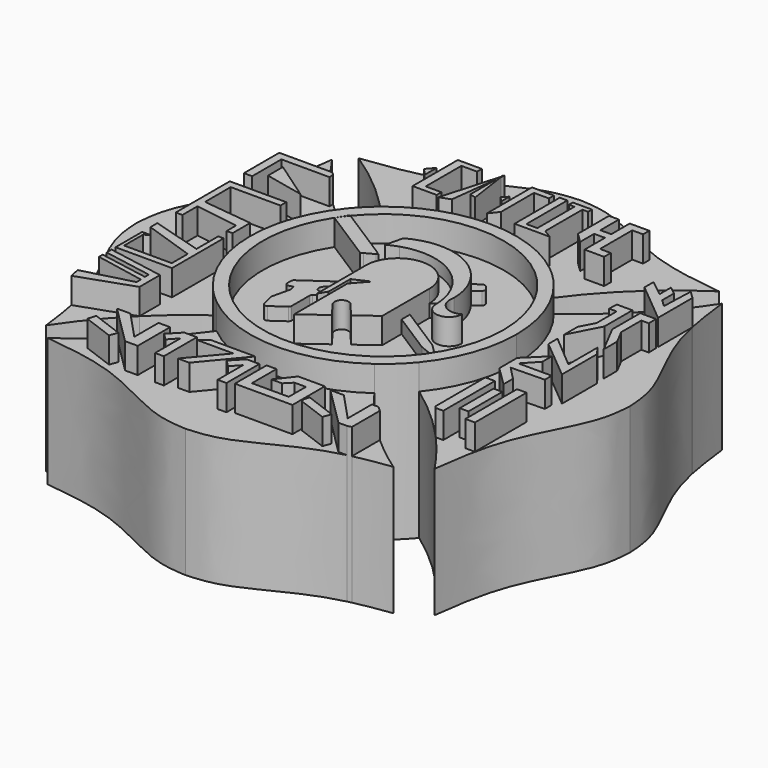
from build123d import *

# Parameters (mm, degrees)
F1_DEPTH = 25.4
F0_W     = 1.7295368016
F0_H     = 8.3469077945
F0_W_2   = 1.8799342215
F0_H_2   = 12.7083547413
F2_DEPTH = 27.94
F3_DEPTH = 30.48


with BuildPart() as f1:
    # F0 (on Top) → F1 (new body)
    with BuildSketch(Plane.XY):
        with BuildLine():
            Line((-9.5434431598, 6.2450544718), (-19.9389753342, 12.8866327357))
            ThreePointArc((-19.9389753342, 12.8866327357), (-6.7178785222, -22.7705544246), (23.7408517253, 0))
            ThreePointArc((23.7408517253, 0), (7.9342600231, 22.3757806239), (-18.437547291, 14.9560987738))
            Line((-18.437547291, 14.9560987738), (-8.1693225853, 8.3958556934))
            Line((-8.1693225853, 8.3958556934), (-7.0434035733, 7.6047051698))
            Line((-7.0434035733, 7.6047051698), (-7.338819981, 7.4440424639))
            Line((-7.338819981, 7.4440424639), (-5.8915200862, 6.5193802761))
            Line((-5.8915200862, 6.5193802761), (-5.6063739329, 6.337203889))
            ThreePointArc((-5.6063739329, 6.337203889), (-5.0978071301, 7.1900943467), (-4.4606007655, 7.951691599))
            Line((-4.4606007655, 7.951691599), (-6.14196317, 11.6369343908))
            ThreePointArc((-6.14196317, 11.6369343908), (-7.2015175666, 11.220879576), (-8.2185240178, 10.709552864))
            Line((-8.2185240178, 10.709552864), (-7.3757171631, 14.1661595553))
            ThreePointArc((-7.3757171631, 14.1661595553), (0.1389586127, 15.6738469109), (7.1075247354, 12.4828346309))
            Line((7.1075247354, 12.4828346309), (8.6497746395, 13.5536975911))
            ThreePointArc((8.6497746395, 13.5536975911), (9.0804497837, 13.6546140229), (9.4635845627, 13.4335417562))
            Line((9.4635845627, 13.4335417562), (10.0592304389, 12.6827814665))
            ThreePointArc((10.0592304389, 12.6827814665), (10.1854985957, 12.2403385238), (9.9619292605, 11.8381990487))
            Line((9.9619292605, 11.8381990487), (8.6400744323, 10.7894523474))
            ThreePointArc((8.6400744323, 10.7894523474), (10.4625836154, 7.3364011169), (11.1228358001, 3.4881327301))
            ThreePointArc((11.1228358001, 3.4881327301), (12.1514474693, 0.3059297611), (15.4842836782, 0.0290534226))
            ThreePointArc((15.4842836782, 0.0290534226), (12.8809521086, -2.5042646054), (10.2800289453, 0.0315260388))
            ThreePointArc((10.2800289453, 0.0315260388), (9.9497055154, 2.7308254028), (9.0397551795, 5.2935038865))
            Line((9.0397551795, 5.2935038865), (6.2511023134, 3.5722714383))
            Line((6.2511023134, 3.5722714383), (6.2511023134, -1.2383925481))
            Line((6.2511023134, -1.2383925481), (15.322001506, -7.0336790136))
            Line((15.322001506, -7.0336790136), (18.4107130058, -10.1001587223))
            Line((18.4107130058, -10.1001587223), (14.3876015009, -8.4962207364))
            Line((14.3876015009, -8.4962207364), (6.2511023134, -3.297910997))
            Line((6.2511023134, -3.297910997), (6.2511023134, -8.0626364797))
            Line((6.2511023134, -8.0626364797), (2.3747377821, -10.9250742877))
            Line((2.3747377821, -10.9250742877), (0, -8.0626364797))
            ThreePointArc((0, -8.0626364797), (-1.929433955, -7.8545272669), (-2.1375431679, -9.7839612218))
            Line((-2.1375431679, -9.7839612218), (0, -12.6786604524))
            Line((0, -12.6786604524), (-4.6690521418, -16.1264454246))
            Line((-4.6690521418, -16.1264454246), (-4.6690521418, -2.9718931764))
            Line((-4.6690521418, -2.9718931764), (-2.1375431679, -0.1181978878))
            Line((-2.1375431679, -0.1181978878), (-5.2554947324, -1.5450455321))
            Line((-5.2554947324, -1.5450455321), (-5.2554947324, -6.8612064933))
            Line((-5.2554947324, -6.8612064933), (-6.2511023134, -8.5651436821))
            Line((-6.2511023134, -8.5651436821), (-6.2511023134, -0.1554940756))
            Line((-6.2511023134, -0.1554940756), (-6.4565095615, -0.2993217791))
            ThreePointArc((-6.4565095615, -0.2993217791), (-6.6782063614, -0.5906114223), (-6.6898507105, -0.9564850842))
            Line((-6.6898507105, -0.9564850842), (-6.3532546104, -2.1378945595))
            ThreePointArc((-6.3532546104, -2.1378945595), (-6.3532532132, -2.467333183), (-6.5268767557, -2.7473058105))
            Line((-6.5268767557, -2.7473058105), (-9.5615380632, -5.5079116557))
            ThreePointArc((-9.5615380632, -5.5079116557), (-9.706817276, -5.7094900403), (-9.7581679001, -5.9526011428))
            Line((-9.7581679001, -5.9526011428), (-9.7581679001, -10.3816536972))
            ThreePointArc((-9.7581679001, -10.3816536972), (-9.8260924812, -10.6592385489), (-10.0145167408, -10.8740952384))
            Line((-10.0145167408, -10.8740952384), (-12.6287511028, -12.7046018453))
            ThreePointArc((-12.6287511028, -12.7046018453), (-13.1802241081, -12.7766817128), (-13.5548146017, -12.365585684))
            Line((-13.5548146017, -12.365585684), (-14.1468444432, -10.1226799809))
            ThreePointArc((-14.1468444432, -10.1226799809), (-14.1666748611, -9.9789061741), (-14.1514706229, -9.8345698165))
            Line((-14.1514706229, -9.8345698165), (-13.3251612392, -6.2401265362))
            ThreePointArc((-13.3251612392, -6.2401265362), (-13.3100853679, -6.0897110613), (-13.3330098084, -5.9402902896))
            Line((-13.3330098084, -5.9402902896), (-13.5587407276, -5.1502324641))
            Line((-13.5587407276, -5.1502324641), (-14.2865060916, -5.3581655283))
            ThreePointArc((-14.2865060916, -5.3581655283), (-14.813673449, -5.260071091), (-15.0528176735, -4.7801356982))
            Line((-15.0528176735, -4.7801356982), (-15.0528176735, -3.89823478))
            ThreePointArc((-15.0528176735, -3.89823478), (-14.9848930924, -3.6206499283), (-14.7964688328, -3.4057932388))
            Line((-14.7964688328, -3.4057932388), (-6.2511023134, 2.5777368149))
            Line((-6.2511023134, 2.5777368149), (-6.2511023134, 3.5722714383))
            ThreePointArc((-6.2511023134, 3.5722714383), (-6.228449268, 4.1039666977), (-6.1606543141, 4.6318083912))
            Line((-6.1606543141, 4.6318083912), (-7.9261528326, 5.7597637848))
            Line((-7.9261528326, 5.7597637848), (-9.0801320579, 6.4970269871))
            Line((-9.0801320579, 6.4970269871), (-9.5434431598, 6.2450544718))
        make_face()
    extrude(amount=F1_DEPTH)


with BuildPart() as f1b:
    # F0 (on Top) → F1, piece 2 (new body)
    with BuildSketch(Plane.XY):
        with BuildLine():
            ThreePointArc((-16.6267062797, 20.2924587669), (0, 26.2341617842), (16.6267062797, 20.2924587669))
            ThreePointArc((16.6267062797, 20.2924587669), (25.2329664201, 30.182800565), (35.5137959123, 38.318593055))
            add(Edge.make_bspline(
                [(35.5137959123, 38.318593055), (30.4620352986, 38.9509589957), (20.4597656889, 40.2030164693), (7.4866494732, 48.2293636919), (2.1728610161, 48.5746910392), (0, 48.7149081634)],
                knots=[0, 0, 0, 0, 0.3760666411, 0.7445958397, 0.9996624927, 0.9996624927, 0.9996624927, 0.9996624927], degree=3))
            add(Edge.make_bspline(
                [(-35.5137959123, 38.318593055), (-30.4620352986, 38.9509589957), (-20.4597656889, 40.2030164693), (-7.4866494732, 48.2293636919), (-2.1728610161, 48.5746910392), (0, 48.7149081634)],
                knots=[0, 0, 0, 0, 0.3760666411, 0.7445958397, 0.9996624927, 0.9996624927, 0.9996624927, 0.9996624927], degree=3))
            ThreePointArc((-35.5137959123, 38.318593055), (-25.2329664201, 30.182800565), (-16.6267062797, 20.2924587669))
        make_face()
        Polygon((-19.3263869733, 34.2127773911), (-18.0286001414, 35.7136428356), (-18.0286001414, 34.2127773911), (-18.0286001414, 32.7141773911), align=None, mode=Mode.SUBTRACT)
        Polygon((-15.4862534255, 39.7773832083), (-12.3972799629, 39.7773832083), (-12.3972799629, 38.6037752032), (-15.4862534255, 38.6037752032), (-15.4862534255, 34.2127773911), (-15.4862534255, 29.8217795789), (-12.3972799629, 29.8217795789), (-12.3972799629, 28.6481715739), (-17.1347092837, 28.6481715739), (-17.1347092837, 34.2127773911), (-17.1347092837, 38.6037752032), (-17.1347092837, 39.7773832083), align=None, mode=Mode.SUBTRACT)
        Polygon((-8.408809687, 39.7450013558), (-8.2768853754, 40.2063913643), (-8.3679740047, 39.4611965301), (-7.2505346718, 31.6950798014), (-8.4751974791, 32.04524516), (-8.4751974791, 38.5840027483), (-9.649637936, 28.9759213881), (-11.7087768862, 28.2037480728), (-8.4751974791, 39.5128177376), (-8.4751974791, 40.2063913643), align=None, mode=Mode.SUBTRACT)
        Polygon((-4.2724665254, 34.2127773911), (-3.2887738198, 35.2003201842), (-3.2887738198, 34.2127773911), (-3.2887738198, 33.2252345979), align=None, mode=Mode.SUBTRACT)
        Polygon((-2.5195907801, 38.5379008949), (-2.5195907801, 39.7773832083), (-1.133499667, 39.7773832083), (1.8175337464, 39.7773832083), (1.8175337464, 38.5379008949), (-1.133499667, 38.5379008949), (-1.133499667, 34.2127773911), (-1.133499667, 30.4379425943), (-2.5195907801, 28.6481715739), (-2.5195907801, 34.2127773911), align=None, mode=Mode.SUBTRACT)
        Polygon((2.9608625919, 29.696483165), (2.9608625919, 39.7773832083), (4.4449735433, 39.7773832083), (4.4449735433, 29.696483165), (6.6135358065, 29.696483165), (6.6135358065, 38.8293154538), (5.534986034, 38.8293154538), (5.534986034, 39.7773832083), (6.6135358065, 39.7773832083), (8.1796292216, 39.7773832083), (9.3080047518, 39.7773832083), (9.3080047518, 38.8293154538), (8.1796292216, 38.8293154538), (8.1796292216, 29.696483165), (9.8721999675, 28.6481715739), (8.1796292216, 28.6481715739), (6.6135358065, 28.6481715739), (4.4449735433, 28.6481715739), (2.9608625919, 28.6481715739), align=None, mode=Mode.SUBTRACT)
        Polygon((12.6640442759, 35.2156497538), (12.6640442759, 39.7773832083), (14.6210510284, 39.7773832083), (14.6210510284, 35.2156497538), (16.7559627444, 35.2156497538), (16.7559627444, 38.2401160896), (16.7559627444, 39.7773832083), (18.4757579118, 39.7773832083), (20.6106770784, 39.7773832083), (20.6106770784, 38.2401160896), (18.4757579118, 38.2401160896), (18.4757579118, 30.2934832871), (20.6106770784, 30.2934832871), (20.6106770784, 28.6481715739), (18.4757579118, 28.6481715739), (16.7559627444, 28.6481715739), (16.7559627444, 30.2934832871), (16.7559627444, 33.6737670004), (14.6210510284, 33.6737670004), (14.6210510284, 30.2341803908), (12.6640442759, 32.1318842471), (12.6640442759, 33.6737670004), align=None, mode=Mode.SUBTRACT)
    extrude(amount=F1_DEPTH)



with BuildPart() as f1c:
    # F0 (on Top) → F1, piece 3 (new body)
    with BuildSketch(Plane.XY):
        with BuildLine():
            ThreePointArc((-20.3356751091, -16.5738215983), (-26.2341617842, 0), (-20.3356751091, 16.5738215983))
            ThreePointArc((-20.3356751091, 16.5738215983), (-24.8128492339, 20.0548614406), (-28.9973442697, 23.8827496081))
            Line((-28.9973442697, 23.8827496081), (-28.9973442697, 22.9817052072))
            Line((-28.9973442697, 22.9817052072), (-38.4649895132, 22.9817052072))
            Line((-38.4649895132, 22.9817052072), (-38.4649895132, 15.7891533872))
            Line((-38.4649895132, 15.7891533872), (-40.0955304503, 15.7891533872))
            Line((-40.0955304503, 15.7891533872), (-40.0955304503, 22.9817052072))
            Line((-40.0955304503, 22.9817052072), (-40.0955304503, 24.4979433319))
            Line((-40.0955304503, 24.4979433319), (-38.4649895132, 24.4979433319))
            Line((-38.4649895132, 24.4979433319), (-29.6104829395, 24.4979433319))
            ThreePointArc((-29.6104829395, 24.4979433319), (-34.2813337884, 29.7377471459), (-38.4109179846, 35.4139189217))
            add(Edge.make_bspline(
                [(-38.4109179846, 35.4139189217), (-39.03013029, 30.3605291582), (-40.2561441291, 20.3550339017), (-48.2486906125, 7.3610662707), (-48.5801831474, 2.0463968131), (-48.7147430824, -0.1268218738)],
                knots=[0, 0, 0, 0, 0.3760666411, 0.7445958397, 0.9996624927, 0.9996624927, 0.9996624927, 0.9996624927], degree=3))
            add(Edge.make_bspline(
                [(-39.9029320846, -25.4186008721), (-40.291396554, -23.7892445191), (-42.1955076013, -17.2767114258), (-48.2097099, -7.6121819354), (-48.5688697193, -2.2993104926), (-48.7147430824, -0.1268218738)],
                knots=[0.2537440472, 0.2537440472, 0.2537440472, 0.2537440472, 0.3760666411, 0.7445958397, 0.9996624927, 0.9996624927, 0.9996624927, 0.9996624927], degree=3))
            Line((-39.9029320846, -25.4186008721), (-30.3178839386, -22.8653751711))
            Line((-30.3178839386, -22.8653751711), (-30.3178839386, -21.7938103179))
            Line((-30.3178839386, -21.7938103179), (-40.0955304503, -19.896445463))
            Line((-40.0955304503, -19.896445463), (-40.0955304503, -18.9949036293))
            Line((-40.0955304503, -18.9949036293), (-30.4072680445, -20.7157038549))
            Line((-30.4072680445, -20.7157038549), (-30.4072680445, -19.7573721554))
            Line((-30.4072680445, -19.7573721554), (-40.0955304503, -18.0365719298))
            Line((-40.0955304503, -18.0365719298), (-40.0955304503, -16.8199502901))
            Line((-40.0955304503, -16.8199502901), (-28.9663188159, -18.7966876129))
            Line((-28.9663188159, -18.7966876129), (-28.9663188159, -23.8520183066))
            ThreePointArc((-28.9663188159, -23.8520183066), (-24.7961597103, -20.0407828139), (-20.3356751091, -16.5738215983))
        make_face()
        Polygon((-39.4113734365, -15.825872908), (-40.0955304503, -15.825872908), (-40.0955304503, -14.5612113575), (-40.0955304503, -9.270174096), (-39.4113734365, -9.270174096), (-38.4338088334, -9.270174096), (-39.4113734365, -9.9116172462), (-39.4113734365, -14.5612113575), (-30.0203710794, -14.5612113575), (-30.0203710794, -10.6391225128), (-40.0955304503, -7.2353460291), (-40.0955304503, -5.5188663701), (-30.0203710794, -8.5023660779), (-30.0203710794, -3.1159945229), (-28.9663188159, -3.1159945229), (-28.9663188159, -15.825872908), (-30.0203710794, -15.825872908), align=None, mode=Mode.SUBTRACT)
        Polygon((-28.9663188159, 3.4426770708), (-28.9663188159, -0.9187736014), (-30.131842941, -0.9187736014), (-30.131842941, 1.4352052734), (-38.7795418501, 2.7206736781), (-38.7795418501, -0.9939648608), (-40.0955304503, -0.9939648608), (-40.0955304503, 2.9162935516), (-40.0955304503, 4.7210327884), (-40.0955304503, 10.8872077962), (-40.0955304503, 12.3159609338), (-38.7795418501, 12.3159609338), (-28.9663188159, 12.3159609338), (-28.9663188159, 10.8872077962), (-38.7795418501, 10.8872077962), (-38.7795418501, 4.569871897), align=None, mode=Mode.SUBTRACT)
        Polygon((-36.6944596171, 21.1480132839), (-28.9663188159, 15.7891533872), (-36.6944596171, 17.4804798862), align=None, mode=Mode.SUBTRACT)
    extrude(amount=F1_DEPTH)


with BuildPart() as f1d:
    # F0 (on Top) → F1, piece 4 (new body)
    with BuildSketch(Plane.XY):
        with BuildLine():
            ThreePointArc((-38.2774990271, -35.2107815006), (-33.9169619408, -29.2895345009), (-28.9663188159, -23.8520183066))
            Line((-28.9663188159, -23.8520183066), (-39.4506689096, -27.5013607093))
            add(Edge.make_bspline(
                [(-38.2774990271, -35.2107815006), (-38.6070013497, -32.6363948006), (-38.9448289643, -30.0626275198), (-39.4506689096, -27.5013607093)],
                knots=[0.0099947999, 0.0099947999, 0.0099947999, 0.0099947999, 0.2017045948, 0.2017045948, 0.2017045948, 0.2017045948], degree=3))
        make_face()
    extrude(amount=F1_DEPTH)


with BuildPart() as f1e:
    # F0 (on Top) → F1, piece 5 (new body)
    with BuildSketch(Plane.XY):
        with BuildLine():
            ThreePointArc((32.9154281705, -38.6499835796), (29.2232816096, -35.9310098419), (25.7146905784, -32.9789676014))
            Line((25.7146905784, -32.9789676014), (25.7146905784, -39.8764228197))
            add(Edge.make_bspline(
                [(32.9154281705, -38.6499835796), (30.5086862404, -38.968303093), (28.1053161528, -39.3335941205), (25.7146905784, -39.8764228197)],
                knots=[0.0644873221, 0.0644873221, 0.0644873221, 0.0644873221, 0.2437419627, 0.2437419627, 0.2437419627, 0.2437419627], degree=3))
        make_face()
    extrude(amount=F1_DEPTH)


with BuildPart() as f1f:
    # F0 (on Top) → F1, piece 6 (new body)
    with BuildSketch(Plane.XY):
        with BuildLine():
            ThreePointArc((20.3356751091, 16.5738215983), (24.7155885558, 8.7960745141), (26.2341617842, 0))
            ThreePointArc((26.2341617842, 0), (24.7155885558, -8.7960745141), (20.3356751091, -16.5738215983))
            ThreePointArc((20.3356751091, -16.5738215983), (26.1532390663, -21.2149239813), (31.4520317335, -26.4405031831))
            Line((31.4520317335, -26.4405031831), (31.4520317335, -14.1721851071))
            Line((31.4520317335, -14.1721851071), (33.331965955, -14.1721851071))
            Line((33.331965955, -14.1721851071), (33.331965955, -26.8805398485))
            Line((33.331965955, -26.8805398485), (31.8503183646, -26.8805398485))
            ThreePointArc((31.8503183646, -26.8805398485), (35.2187146617, -30.9262204528), (38.2774990271, -35.2107815006))
            add(Edge.make_bspline(
                [(38.2774990271, -35.2107815006), (38.9066871287, -30.2949634039), (40.2302025567, -20.4348606893), (48.2097099, -7.6121819354), (48.5688697193, -2.2993104926), (48.7147430824, -0.1268218738)],
                knots=[0.0099947999, 0.0099947999, 0.0099947999, 0.0099947999, 0.3760666411, 0.7445958397, 0.9996624927, 0.9996624927, 0.9996624927, 0.9996624927], degree=3))
            add(Edge.make_bspline(
                [(39.7814951576, 26.3571659412), (40.2034923324, 24.3406530333), (42.055934891, 17.4290048881), (48.2486906125, 7.3610662707), (48.5801831474, 2.0463968131), (48.7147430824, -0.1268218738)],
                knots=[0.2251076454, 0.2251076454, 0.2251076454, 0.2251076454, 0.3760666411, 0.7445958397, 0.9996624927, 0.9996624927, 0.9996624927, 0.9996624927], degree=3))
            Line((39.7814951576, 26.3571659412), (39.7814951576, 17.9630034724))
            Line((39.7814951576, 17.9630034724), (31.8105734624, 24.5803744653))
            Line((31.8105734624, 24.5803744653), (31.8105734624, 26.8362947861))
            ThreePointArc((31.8105734624, 26.8362947861), (26.3526094356, 21.3925542151), (20.3356751091, 16.5738215983))
        make_face()
        with Locations((35.6254874933, -20.4511656305)):
            Rectangle(F0_W, F0_H, mode=Mode.SUBTRACT)
        with Locations((38.6333837379, -20.5263624778)):
            Rectangle(F0_W_2, F0_H_2, mode=Mode.SUBTRACT)
        Polygon((35.0392975564, -14.1721851071), (31.2011621612, -10.4123166641), (31.2011621612, -6.0132703623), (35.0392975564, -2.2534056445), (35.0392975564, -4.58452095), (32.4795174132, -7.3292254349), (39.0592871885, -7.3292254349), (39.0592871885, -9.0211666068), (32.4419185239, -9.1715603014), (35.0392975564, -11.8410660764), align=None, mode=Mode.SUBTRACT)
        Polygon((32.0551983751, 0.6040969053), (32.0551983751, 2.8600209514), (38.7086647675, -2.7797854384), (38.7086647675, 4.3910338258), (40.0261200704, 2.6344248215), (40.0261200704, -6.0132703623), align=None, mode=Mode.SUBTRACT)
        Polygon((32.0020235814, 15.6471395055), (32.0551983751, 17.4550079862), (35.1392060257, 17.4550079862), (35.1392060257, 10.5691590468), (32.0020235814, 4.534069554), (32.0020235814, 7.8573563257), (33.4837888663, 10.7078714808), (33.4837888663, 15.6471395055), align=None, mode=Mode.SUBTRACT)
        Polygon((36.6812079884, 17.4550079862), (39.765215639, 17.4550079862), (39.8183904327, 15.6471395055), (38.3366251478, 15.6471395055), (38.3366251478, 10.7078714808), (39.8183904327, 7.8573563257), (39.8183904327, 4.534069554), (36.6812079884, 10.5691590468), align=None, mode=Mode.SUBTRACT)
    extrude(amount=F1_DEPTH)


with BuildPart() as f1g:
    # F0 (on Top) → F1, piece 7 (new body)
    with BuildSketch(Plane.XY):
        with BuildLine():
            ThreePointArc((38.4109179846, 35.4139189217), (35.2747322236, 30.998921866), (31.8105734624, 26.8362947861))
            Line((31.8105734624, 26.8362947861), (35.0440621115, 24.2795852134))
            Line((35.0440621115, 24.2795852134), (35.0440621115, 27.0618871907))
            Line((35.0440621115, 27.0618871907), (36.6232052185, 25.8587283203))
            Line((36.6232052185, 25.8587283203), (36.6232052185, 22.9260326484))
            Line((36.6232052185, 22.9260326484), (38.051958356, 21.5724800835))
            Line((38.051958356, 21.5724800835), (38.2775470354, 27.8890580991))
            Line((38.2775470354, 27.8890580991), (39.7547533603, 26.4857115416))
            add(Edge.make_bspline(
                [(38.4109179846, 35.4139189217), (38.7762876513, 32.4321381698), (39.141657318, 29.4503574178), (39.7547533603, 26.4857115416)],
                knots=[0, 0, 0, 0, 0.2219002144, 0.2219002144, 0.2219002144, 0.2219002144], degree=3))
        make_face()
    extrude(amount=F1_DEPTH)


with BuildPart() as f1h:
    # F0 (on Top) → F1, piece 8 (new body)
    with BuildSketch(Plane.XY):
        with BuildLine():
            Line((15.4275732894, -21.4819234181), (15.3033273432, -21.3082006924))
            ThreePointArc((15.3033273432, -21.3082006924), (-0.8341258102, -26.2208977468), (-16.6267062797, -20.2924587669))
            ThreePointArc((-16.6267062797, -20.2924587669), (-21.4138621586, -26.2442472283), (-26.8137526248, -31.6462681696))
            Line((-26.8137526248, -31.6462681696), (-24.5010119255, -31.6462681696))
            Line((-24.5010119255, -31.6462681696), (-19.1837486203, -37.3357331448))
            Line((-19.1837486203, -37.3357331448), (-19.1837486203, -31.3804053769))
            Line((-19.1837486203, -31.3804053769), (-16.8973293479, -31.3804053769))
            Line((-16.8973293479, -31.3804053769), (-16.8973293479, -39.3562905558))
            Line((-16.8973293479, -39.3562905558), (-19.3964403446, -39.3562905558))
            Line((-19.3964403446, -39.3562905558), (-26.995701496, -31.8090835655))
            ThreePointArc((-26.995701496, -31.8090835655), (-31.1314824425, -35.2251398118), (-35.5137959123, -38.318593055))
            add(Edge.make_bspline(
                [(-35.5137959123, -38.318593055), (-30.4620352986, -38.9509589957), (-20.4597656889, -40.2030164693), (-7.4866494732, -48.2293636919), (-2.1728610161, -48.5746910392), (0, -48.7149081634)],
                knots=[0, 0, 0, 0, 0.3760666411, 0.7445958397, 0.9996624927, 0.9996624927, 0.9996624927, 0.9996624927], degree=3))
            add(Edge.make_bspline(
                [(24.9123165873, -40.065583976), (23.4170540138, -40.4314467219), (17.0361868562, -42.3211530834), (7.4866494732, -48.2293636919), (2.1728610161, -48.5746910392), (0, -48.7149081634)],
                knots=[0.263808887, 0.263808887, 0.263808887, 0.263808887, 0.3760666411, 0.7445958397, 0.9996624927, 0.9996624927, 0.9996624927, 0.9996624927], degree=3))
            Line((24.9123165873, -40.065583976), (23.2155795817, -40.065583976))
            Line((23.2155795817, -40.065583976), (15.4523800735, -32.3555615898))
            Line((15.4523800735, -32.3555615898), (18.1110080008, -32.3555615898))
            Line((18.1110080008, -32.3555615898), (23.428271306, -38.045026565))
            Line((23.428271306, -38.045026565), (23.428271306, -32.0896987971))
            Line((23.428271306, -32.0896987971), (24.7429571153, -32.0896987971))
            ThreePointArc((24.7429571153, -32.0896987971), (19.8204675296, -27.0183473246), (15.4275732894, -21.4819234181))
        make_face()
        Polygon((-28.6157503724, -37.1411293745), (-28.1167414363, -35.5278660611), (-21.948726135, -37.8142862648), (-22.5347847712, -39.3952811446), align=None, mode=Mode.SUBTRACT)
        Polygon((-14.9043574929, -35.0307189029), (-16.2579119205, -33.6771644752), (-14.0771865845, -31.4212441545), (-11.5956738591, -31.4212441545), (-11.5956738591, -39.5425595444), (-13.325214386, -39.5425595444), (-13.325214386, -33.301178376), align=None, mode=Mode.SUBTRACT)
        Polygon((-7.1978791382, -38.7864187358), (-9.4538031842, -38.7864187358), (-3.8139967944, -32.1329523434), (-10.9848160587, -32.1329523434), (-9.2282070543, -30.8154970406), (-0.5805118706, -30.8154970406), align=None, mode=Mode.SUBTRACT)
        Polygon((-1.8102118192, -35.9862744808), (-3.1637662469, -34.6327200532), (-0.9830409108, -32.3767997324), (1.4984718146, -32.3767997324), (1.4984718146, -40.4981151223), (-0.2310687123, -40.4981151223), (-0.2310687123, -34.256733954), align=None, mode=Mode.SUBTRACT)
        Polygon((14.1554349825, -37.335851355), (14.49527849, -36.2371594813), (20.6632937913, -38.523579685), (20.0772351551, -40.1045745648), (14.4032866999, -38.001299889), align=None, mode=Mode.SUBTRACT)
        Polygon((2.6414692402, -39.8631114613), (2.6414692402, -32.0426062781), (4.5965984464, -32.0426062781), (4.5965984464, -38.0959943969), (11.8531472981, -38.0959943969), (11.8531472981, -33.8699700235), (9.5842894095, -33.8699700235), (8.2436725497, -35.2384937096), (6.1381459236, -35.2384937096), (8.7700523436, -31.8922107208), (13.9962695539, -31.8922107208), (13.9962695539, -39.8631114613), align=None, mode=Mode.SUBTRACT)
    extrude(amount=F1_DEPTH)


with BuildPart() as f1i:
    # F0 (on Top) → F1, piece 9 (new body)
    with BuildSketch(Plane.XY):
        with BuildLine():
            add(Edge.make_bspline(
                [(-7.2091906331, -1.5097639989), (-8.2920949454, 0.046911573), (-9.9321888534, -2.2490228676), (-11.5722827613, -4.5449573081), (-8.8492845411, -3.8056984394), (-6.1262863209, -3.0664395708), (-7.2091906331, -1.5097639989)],
                knots=[0, 0, 0, 2.0943951024, 2.0943951024, 4.1887902048, 4.1887902048, 6.2831853072, 6.2831853072, 6.2831853072], degree=2, weights=[1, 0.5, 1, 0.5, 1, 0.5, 1]))
        make_face()
    extrude(amount=F1_DEPTH)

    # F0 (on Top) → F2 (join)
    with BuildSketch(Plane.XY):
        with BuildLine():
            Line((-6.2511023134, -0.1554940756), (-6.2511023134, 2.5777368149))
            Line((-6.2511023134, 2.5777368149), (-14.7964688328, -3.4057932388))
            ThreePointArc((-14.7964688328, -3.4057932388), (-14.9848930924, -3.6206499283), (-15.0528176735, -3.89823478))
            Line((-15.0528176735, -3.89823478), (-15.0528176735, -4.7801356982))
            ThreePointArc((-15.0528176735, -4.7801356982), (-14.813673449, -5.260071091), (-14.2865060916, -5.3581655283))
            Line((-14.2865060916, -5.3581655283), (-13.5587407276, -5.1502324641))
            Line((-13.5587407276, -5.1502324641), (-13.3330098084, -5.9402902896))
            ThreePointArc((-13.3330098084, -5.9402902896), (-13.3100853679, -6.0897110613), (-13.3251612392, -6.2401265362))
            Line((-13.3251612392, -6.2401265362), (-14.1514706229, -9.8345698165))
            ThreePointArc((-14.1514706229, -9.8345698165), (-14.1666748611, -9.9789061741), (-14.1468444432, -10.1226799809))
            Line((-14.1468444432, -10.1226799809), (-13.5548146017, -12.365585684))
            ThreePointArc((-13.5548146017, -12.365585684), (-13.1802241081, -12.7766817128), (-12.6287511028, -12.7046018453))
            Line((-12.6287511028, -12.7046018453), (-10.0145167408, -10.8740952384))
            ThreePointArc((-10.0145167408, -10.8740952384), (-9.8260924812, -10.6592385489), (-9.7581679001, -10.3816536972))
            Line((-9.7581679001, -10.3816536972), (-9.7581679001, -5.9526011428))
            ThreePointArc((-9.7581679001, -5.9526011428), (-9.706817276, -5.7094900403), (-9.5615380632, -5.5079116557))
            Line((-9.5615380632, -5.5079116557), (-6.5268767557, -2.7473058105))
            ThreePointArc((-6.5268767557, -2.7473058105), (-6.3532532132, -2.467333183), (-6.3532546104, -2.1378945595))
            Line((-6.3532546104, -2.1378945595), (-6.6898507105, -0.9564850842))
            ThreePointArc((-6.6898507105, -0.9564850842), (-6.6782063614, -0.5906114223), (-6.4565095615, -0.2993217791))
            Line((-6.4565095615, -0.2993217791), (-6.2511023134, -0.1554940756))
        make_face()
        with BuildLine():
            add(Edge.make_bspline(
                [(-7.2091906331, -1.5097639989), (-8.2920949454, 0.046911573), (-9.9321888534, -2.2490228676), (-11.5722827613, -4.5449573081), (-8.8492845411, -3.8056984394), (-6.1262863209, -3.0664395708), (-7.2091906331, -1.5097639989)],
                knots=[0, 0, 0, 2.0943951024, 2.0943951024, 4.1887902048, 4.1887902048, 6.2831853072, 6.2831853072, 6.2831853072], degree=2, weights=[1, 0.5, 1, 0.5, 1, 0.5, 1]))
        make_face(mode=Mode.SUBTRACT)
    extrude(amount=F2_DEPTH)



with BuildPart() as f2:
    # F0 (on Top) → F2, piece 2 (new body)
    with BuildSketch(Plane.XY):
        with BuildLine():
            Line((-7.338819981, 7.4440424639), (-9.0801320579, 6.4970269871))
            Line((-9.0801320579, 6.4970269871), (-7.9261528326, 5.7597637848))
            Line((-7.9261528326, 5.7597637848), (-6.1606543141, 4.6318083912))
            ThreePointArc((-6.1606543141, 4.6318083912), (-5.9449837588, 5.5044847392), (-5.6063739329, 6.337203889))
            Line((-5.6063739329, 6.337203889), (-5.8915200862, 6.5193802761))
            Line((-5.8915200862, 6.5193802761), (-7.338819981, 7.4440424639))
        make_face()
    extrude(amount=F2_DEPTH)


with BuildPart() as f2b:
    # F0 (on Top) → F2, piece 3 (new body)
    with BuildSketch(Plane.XY):
        Polygon((15.322001506, -7.0336790136), (6.2511023134, -1.2383925481), (6.2511023134, -3.297910997), (14.3876015009, -8.4962207364), (18.4107130058, -10.1001587223), align=None)
    extrude(amount=F2_DEPTH)


with BuildPart() as f2c:
    # F0 (on Top) → F2, piece 4 (new body)
    with BuildSketch(Plane.XY):
        with BuildLine():
            Line((-6.14196317, 11.6369343908), (-4.4606007655, 7.951691599))
            ThreePointArc((-4.4606007655, 7.951691599), (2.3656509007, 9.3584598165), (6.2511023134, 3.5722714383))
            Line((6.2511023134, 3.5722714383), (9.0397551795, 5.2935038865))
            ThreePointArc((9.0397551795, 5.2935038865), (2.6501831797, 11.3402571067), (-6.14196317, 11.6369343908))
        make_face()
    extrude(amount=F2_DEPTH)


with BuildPart() as f2d:
    # F0 (on Top) → F2, piece 5 (new body)
    with BuildSketch(Plane.XY):
        with BuildLine():
            Line((8.6497746395, 13.5536975911), (7.1075247354, 12.4828346309))
            ThreePointArc((7.1075247354, 12.4828346309), (7.9128114811, 11.6714501485), (8.6400744323, 10.7894523474))
            Line((8.6400744323, 10.7894523474), (9.9619292605, 11.8381990487))
            ThreePointArc((9.9619292605, 11.8381990487), (10.1854985957, 12.2403385238), (10.0592304389, 12.6827814665))
            Line((10.0592304389, 12.6827814665), (9.4635845627, 13.4335417562))
            ThreePointArc((9.4635845627, 13.4335417562), (9.0804497837, 13.6546140229), (8.6497746395, 13.5536975911))
        make_face()
    extrude(amount=F2_DEPTH)


with BuildPart() as f1i_1:
    add(f1i.part)

    add(f2.part)  # F3 merges F2

    add(f2b.part)  # F3 merges F2b

    add(f2c.part)  # F3 merges F2c
    # F0 (on Top) → F3 (join)
    with BuildSketch(Plane.XY):
        with BuildLine():
            ThreePointArc((-18.437547291, 14.9560987738), (-19.2161402113, 13.9415923057), (-19.9389753342, 12.8866327357))
            Line((-19.9389753342, 12.8866327357), (-9.5434431598, 6.2450544718))
            Line((-9.5434431598, 6.2450544718), (-8.1693225853, 8.3958556934))
            Line((-8.1693225853, 8.3958556934), (-18.437547291, 14.9560987738))
        make_face()
        Polygon((-8.1693225853, 8.3958556934), (-9.5434431598, 6.2450544718), (-9.0801320579, 6.4970269871), (-7.338819981, 7.4440424639), (-7.0434035733, 7.6047051698), align=None)
        with BuildLine():
            ThreePointArc((-5.6063739329, 6.337203889), (-5.9449837588, 5.5044847392), (-6.1606543141, 4.6318083912))
            ThreePointArc((-6.1606543141, 4.6318083912), (-6.228449268, 4.1039666977), (-6.2511023134, 3.5722714383))
            Line((-6.2511023134, 3.5722714383), (-6.2511023134, 2.5777368149))
            Line((-6.2511023134, 2.5777368149), (-6.2511023134, -0.1554940756))
            Line((-6.2511023134, -0.1554940756), (-6.2511023134, -8.5651436821))
            Line((-6.2511023134, -8.5651436821), (-5.2554947324, -6.8612064933))
            Line((-5.2554947324, -6.8612064933), (-5.2554947324, -1.5450455321))
            Line((-5.2554947324, -1.5450455321), (-2.1375431679, -0.1181978878))
            Line((-2.1375431679, -0.1181978878), (-4.6690521418, -2.9718931764))
            Line((-4.6690521418, -2.9718931764), (-4.6690521418, -16.1264454246))
            Line((-4.6690521418, -16.1264454246), (0, -12.6786604524))
            Line((0, -12.6786604524), (-2.1375431679, -9.7839612218))
            ThreePointArc((-2.1375431679, -9.7839612218), (-1.929433955, -7.8545272669), (0, -8.0626364797))
            Line((0, -8.0626364797), (2.3747377821, -10.9250742877))
            Line((2.3747377821, -10.9250742877), (6.2511023134, -8.0626364797))
            Line((6.2511023134, -8.0626364797), (6.2511023134, -3.297910997))
            Line((6.2511023134, -3.297910997), (6.2511023134, -1.2383925481))
            Line((6.2511023134, -1.2383925481), (6.2511023134, 3.5722714383))
            ThreePointArc((6.2511023134, 3.5722714383), (2.3656509007, 9.3584598165), (-4.4606007655, 7.951691599))
            ThreePointArc((-4.4606007655, 7.951691599), (-5.0978071301, 7.1900943467), (-5.6063739329, 6.337203889))
        make_face()
        with BuildLine():
            ThreePointArc((-8.2185240178, 10.709552864), (-7.2015175666, 11.220879576), (-6.14196317, 11.6369343908))
            ThreePointArc((-6.14196317, 11.6369343908), (2.6501831797, 11.3402571067), (9.0397551795, 5.2935038865))
            ThreePointArc((9.0397551795, 5.2935038865), (9.9497055154, 2.7308254028), (10.2800289453, 0.0315260388))
            ThreePointArc((10.2800289453, 0.0315260388), (12.8809521086, -2.5042646054), (15.4842836782, 0.0290534226))
            ThreePointArc((15.4842836782, 0.0290534226), (12.1514474693, 0.3059297611), (11.1228358001, 3.4881327301))
            ThreePointArc((11.1228358001, 3.4881327301), (10.4625836154, 7.3364011169), (8.6400744323, 10.7894523474))
            ThreePointArc((8.6400744323, 10.7894523474), (7.9128114811, 11.6714501485), (7.1075247354, 12.4828346309))
            ThreePointArc((7.1075247354, 12.4828346309), (0.1389586127, 15.6738469109), (-7.3757171631, 14.1661595553))
            Line((-7.3757171631, 14.1661595553), (-8.2185240178, 10.709552864))
        make_face()
    extrude(amount=F3_DEPTH)


with BuildPart() as f1b_1:
    add(f1b.part)

    add(f1c.part)  # F3#2 merges F1c

    add(f1d.part)  # F3#2 merges F1d

    add(f1e.part)  # F3#2 merges F1e

    add(f1f.part)  # F3#2 merges F1f

    add(f1g.part)  # F3#2 merges F1g

    add(f1h.part)  # F3#2 merges F1h
    # F0 (on Top) → F3, piece 2 (join)
    with BuildSketch(Plane.XY):
        with BuildLine():
            Line((-28.9973442697, 22.9817052072), (-28.9973442697, 23.8827496081))
            ThreePointArc((-28.9973442697, 23.8827496081), (-29.3048560825, 24.1894071405), (-29.6104829395, 24.4979433319))
            Line((-29.6104829395, 24.4979433319), (-38.4649895132, 24.4979433319))
            Line((-38.4649895132, 24.4979433319), (-40.0955304503, 24.4979433319))
            Line((-40.0955304503, 24.4979433319), (-40.0955304503, 22.9817052072))
            Line((-40.0955304503, 22.9817052072), (-40.0955304503, 15.7891533872))
            Line((-40.0955304503, 15.7891533872), (-38.4649895132, 15.7891533872))
            Line((-38.4649895132, 15.7891533872), (-38.4649895132, 22.9817052072))
            Line((-38.4649895132, 22.9817052072), (-28.9973442697, 22.9817052072))
        make_face()
        Polygon((-36.6944596171, 17.4804798862), (-28.9663188159, 15.7891533872), (-36.6944596171, 21.1480132839), align=None)
        Polygon((-40.0955304503, -14.5612113575), (-40.0955304503, -15.825872908), (-39.4113734365, -15.825872908), (-30.0203710794, -15.825872908), (-28.9663188159, -15.825872908), (-28.9663188159, -3.1159945229), (-30.0203710794, -3.1159945229), (-30.0203710794, -8.5023660779), (-40.0955304503, -5.5188663701), (-40.0955304503, -7.2353460291), (-30.0203710794, -10.6391225128), (-30.0203710794, -14.5612113575), (-39.4113734365, -14.5612113575), (-39.4113734365, -9.9116172462), (-38.4338088334, -9.270174096), (-39.4113734365, -9.270174096), (-40.0955304503, -9.270174096), align=None)
        with BuildLine():
            Line((-39.4506689096, -27.5013607093), (-28.9663188159, -23.8520183066))
            Line((-28.9663188159, -23.8520183066), (-28.9663188159, -18.7966876129))
            Line((-28.9663188159, -18.7966876129), (-40.0955304503, -16.8199502901))
            Line((-40.0955304503, -16.8199502901), (-40.0955304503, -18.0365719298))
            Line((-40.0955304503, -18.0365719298), (-30.4072680445, -19.7573721554))
            Line((-30.4072680445, -19.7573721554), (-30.4072680445, -20.7157038549))
            Line((-30.4072680445, -20.7157038549), (-40.0955304503, -18.9949036293))
            Line((-40.0955304503, -18.9949036293), (-40.0955304503, -19.896445463))
            Line((-40.0955304503, -19.896445463), (-30.3178839386, -21.7938103179))
            Line((-30.3178839386, -21.7938103179), (-30.3178839386, -22.8653751711))
            Line((-30.3178839386, -22.8653751711), (-39.9029320846, -25.4186008721))
            add(Edge.make_bspline(
                [(-39.4506689096, -27.5013607093), (-39.5879787104, -26.8061071244), (-39.7376684354, -26.1117746319), (-39.9029320846, -25.4186008721)],
                knots=[0.2017045948, 0.2017045948, 0.2017045948, 0.2017045948, 0.2537440472, 0.2537440472, 0.2537440472, 0.2537440472], degree=3))
        make_face()
        Polygon((-30.131842941, -0.9187736014), (-28.9663188159, -0.9187736014), (-28.9663188159, 3.4426770708), (-38.7795418501, 4.569871897), (-38.7795418501, 10.8872077962), (-28.9663188159, 10.8872077962), (-28.9663188159, 12.3159609338), (-38.7795418501, 12.3159609338), (-40.0955304503, 12.3159609338), (-40.0955304503, 10.8872077962), (-40.0955304503, 4.7210327884), (-40.0955304503, 2.9162935516), (-40.0955304503, -0.9939648608), (-38.7795418501, -0.9939648608), (-38.7795418501, 2.7206736781), (-30.131842941, 1.4352052734), align=None)
        Polygon((-12.3972799629, 38.6037752032), (-12.3972799629, 39.7773832083), (-15.4862534255, 39.7773832083), (-17.1347092837, 39.7773832083), (-17.1347092837, 38.6037752032), (-17.1347092837, 34.2127773911), (-17.1347092837, 28.6481715739), (-12.3972799629, 28.6481715739), (-12.3972799629, 29.8217795789), (-15.4862534255, 29.8217795789), (-15.4862534255, 34.2127773911), (-15.4862534255, 38.6037752032), align=None)
        Polygon((-18.0286001414, 34.2127773911), (-18.0286001414, 35.7136428356), (-19.3263869733, 34.2127773911), (-18.0286001414, 32.7141773911), align=None)
        Polygon((-8.3679740047, 39.4611965301), (-8.2768853754, 40.2063913643), (-8.408809687, 39.7450013558), (-8.4751974791, 40.2063913643), (-8.4751974791, 39.5128177376), (-11.7087768862, 28.2037480728), (-9.649637936, 28.9759213881), (-8.4751974791, 38.5840027483), (-8.4751974791, 32.04524516), (-7.2505346718, 31.6950798014), align=None)
        Polygon((-1.133499667, 39.7773832083), (-2.5195907801, 39.7773832083), (-2.5195907801, 38.5379008949), (-2.5195907801, 34.2127773911), (-2.5195907801, 28.6481715739), (-1.133499667, 30.4379425943), (-1.133499667, 34.2127773911), (-1.133499667, 38.5379008949), (1.8175337464, 38.5379008949), (1.8175337464, 39.7773832083), align=None)
        Polygon((-3.2887738198, 34.2127773911), (-3.2887738198, 35.2003201842), (-4.2724665254, 34.2127773911), (-3.2887738198, 33.2252345979), align=None)
        Polygon((4.4449735433, 39.7773832083), (2.9608625919, 39.7773832083), (2.9608625919, 29.696483165), (2.9608625919, 28.6481715739), (4.4449735433, 28.6481715739), (6.6135358065, 28.6481715739), (8.1796292216, 28.6481715739), (9.8721999675, 28.6481715739), (8.1796292216, 29.696483165), (8.1796292216, 38.8293154538), (9.3080047518, 38.8293154538), (9.3080047518, 39.7773832083), (8.1796292216, 39.7773832083), (6.6135358065, 39.7773832083), (5.534986034, 39.7773832083), (5.534986034, 38.8293154538), (6.6135358065, 38.8293154538), (6.6135358065, 29.696483165), (4.4449735433, 29.696483165), align=None)
        Polygon((14.6210510284, 39.7773832083), (12.6640442759, 39.7773832083), (12.6640442759, 35.2156497538), (12.6640442759, 33.6737670004), (12.6640442759, 32.1318842471), (14.6210510284, 30.2341803908), (14.6210510284, 33.6737670004), (16.7559627444, 33.6737670004), (16.7559627444, 30.2934832871), (16.7559627444, 28.6481715739), (18.4757579118, 28.6481715739), (20.6106770784, 28.6481715739), (20.6106770784, 30.2934832871), (18.4757579118, 30.2934832871), (18.4757579118, 38.2401160896), (20.6106770784, 38.2401160896), (20.6106770784, 39.7773832083), (18.4757579118, 39.7773832083), (16.7559627444, 39.7773832083), (16.7559627444, 38.2401160896), (16.7559627444, 35.2156497538), (14.6210510284, 35.2156497538), align=None)
        with Locations((38.6333837379, -20.5263624778)):
            Rectangle(F0_W_2, F0_H_2)
        with Locations((35.6254874933, -20.4511656305)):
            Rectangle(F0_W, F0_H)
        with BuildLine():
            Line((31.4520317335, -14.1721851071), (31.4520317335, -26.4405031831))
            ThreePointArc((31.4520317335, -26.4405031831), (31.6516357073, -26.6601045641), (31.8503183646, -26.8805398485))
            Line((31.8503183646, -26.8805398485), (33.331965955, -26.8805398485))
            Line((33.331965955, -26.8805398485), (33.331965955, -14.1721851071))
            Line((33.331965955, -14.1721851071), (31.4520317335, -14.1721851071))
        make_face()
        Polygon((31.2011621612, -6.0132703623), (31.2011621612, -10.4123166641), (35.0392975564, -14.1721851071), (35.0392975564, -11.8410660764), (32.4419185239, -9.1715603014), (39.0592871885, -9.0211666068), (39.0592871885, -7.3292254349), (32.4795174132, -7.3292254349), (35.0392975564, -4.58452095), (35.0392975564, -2.2534056445), align=None)
        Polygon((38.7086647675, -2.7797854384), (32.0551983751, 2.8600209514), (32.0551983751, 0.6040969053), (40.0261200704, -6.0132703623), (40.0261200704, 2.6344248215), (38.7086647675, 4.3910338258), align=None)
        Polygon((35.1392060257, 17.4550079862), (32.0551983751, 17.4550079862), (32.0020235814, 15.6471395055), (33.4837888663, 15.6471395055), (33.4837888663, 10.7078714808), (32.0020235814, 7.8573563257), (32.0020235814, 4.534069554), (35.1392060257, 10.5691590468), align=None)
        with BuildLine():
            Line((35.0440621115, 24.2795852134), (31.8105734624, 26.8362947861))
            Line((31.8105734624, 26.8362947861), (31.8105734624, 24.5803744653))
            Line((31.8105734624, 24.5803744653), (39.7814951576, 17.9630034724))
            Line((39.7814951576, 17.9630034724), (39.7814951576, 26.3571659412))
            add(Edge.make_bspline(
                [(39.7547533603, 26.4857115416), (39.7636152861, 26.4428594109), (39.7725289692, 26.4000108602), (39.7814951576, 26.3571659412)],
                knots=[0.2219002144, 0.2219002144, 0.2219002144, 0.2219002144, 0.2251076454, 0.2251076454, 0.2251076454, 0.2251076454], degree=3))
            Line((39.7547533603, 26.4857115416), (38.2775470354, 27.8890580991))
            Line((38.2775470354, 27.8890580991), (38.051958356, 21.5724800835))
            Line((38.051958356, 21.5724800835), (36.6232052185, 22.9260326484))
            Line((36.6232052185, 22.9260326484), (36.6232052185, 25.8587283203))
            Line((36.6232052185, 25.8587283203), (35.0440621115, 27.0618871907))
            Line((35.0440621115, 27.0618871907), (35.0440621115, 24.2795852134))
        make_face()
        Polygon((39.8183904327, 15.6471395055), (39.765215639, 17.4550079862), (36.6812079884, 17.4550079862), (36.6812079884, 10.5691590468), (39.8183904327, 4.534069554), (39.8183904327, 7.8573563257), (38.3366251478, 10.7078714808), (38.3366251478, 15.6471395055), align=None)
        Polygon((-3.8139967944, -32.1329523434), (-9.4538031842, -38.7864187358), (-7.1978791382, -38.7864187358), (-0.5805118706, -30.8154970406), (-9.2282070543, -30.8154970406), (-10.9848160587, -32.1329523434), align=None)
        Polygon((-14.0771865845, -31.4212441545), (-16.2579119205, -33.6771644752), (-14.9043574929, -35.0307189029), (-13.325214386, -33.301178376), (-13.325214386, -39.5425595444), (-11.5956738591, -39.5425595444), (-11.5956738591, -31.4212441545), align=None)
        with BuildLine():
            Line((-24.5010119255, -31.6462681696), (-26.8137526248, -31.6462681696))
            ThreePointArc((-26.8137526248, -31.6462681696), (-26.9046569432, -31.7277542246), (-26.995701496, -31.8090835655))
            Line((-26.995701496, -31.8090835655), (-19.3964403446, -39.3562905558))
            Line((-19.3964403446, -39.3562905558), (-16.8973293479, -39.3562905558))
            Line((-16.8973293479, -39.3562905558), (-16.8973293479, -31.3804053769))
            Line((-16.8973293479, -31.3804053769), (-19.1837486203, -31.3804053769))
            Line((-19.1837486203, -31.3804053769), (-19.1837486203, -37.3357331448))
            Line((-19.1837486203, -37.3357331448), (-24.5010119255, -31.6462681696))
        make_face()
        Polygon((-21.948726135, -37.8142862648), (-28.1167414363, -35.5278660611), (-28.6157503724, -37.1411293745), (-22.5347847712, -39.3952811446), align=None)
        Polygon((-0.9830409108, -32.3767997324), (-3.1637662469, -34.6327200532), (-1.8102118192, -35.9862744808), (-0.2310687123, -34.256733954), (-0.2310687123, -40.4981151223), (1.4984718146, -40.4981151223), (1.4984718146, -32.3767997324), align=None)
        Polygon((4.5965984464, -32.0426062781), (2.6414692402, -32.0426062781), (2.6414692402, -39.8631114613), (13.9962695539, -39.8631114613), (13.9962695539, -31.8922107208), (8.7700523436, -31.8922107208), (6.1381459236, -35.2384937096), (8.2436725497, -35.2384937096), (9.5842894095, -33.8699700235), (11.8531472981, -33.8699700235), (11.8531472981, -38.0959943969), (4.5965984464, -38.0959943969), align=None)
        Polygon((20.6632937913, -38.523579685), (14.49527849, -36.2371594813), (14.1554349825, -37.335851355), (14.4032866999, -38.001299889), (20.0772351551, -40.1045745648), align=None)
        with BuildLine():
            ThreePointArc((25.7146905784, -32.9789676014), (25.2267577343, -32.5365909088), (24.7429571153, -32.0896987971))
            Line((24.7429571153, -32.0896987971), (23.428271306, -32.0896987971))
            Line((23.428271306, -32.0896987971), (23.428271306, -38.045026565))
            Line((23.428271306, -38.045026565), (18.1110080008, -32.3555615898))
            Line((18.1110080008, -32.3555615898), (15.4523800735, -32.3555615898))
            Line((15.4523800735, -32.3555615898), (23.2155795817, -40.065583976))
            Line((23.2155795817, -40.065583976), (24.9123165873, -40.065583976))
            add(Edge.make_bspline(
                [(25.7146905784, -39.8764228197), (25.447068484, -39.9371905765), (25.1796061039, -40.0001832375), (24.9123165873, -40.065583976)],
                knots=[0.2437419627, 0.2437419627, 0.2437419627, 0.2437419627, 0.263808887, 0.263808887, 0.263808887, 0.263808887], degree=3))
            Line((25.7146905784, -39.8764228197), (25.7146905784, -32.9789676014))
        make_face()
        with BuildLine():
            ThreePointArc((20.3356751091, -16.5738215983), (24.7155885558, -8.7960745141), (26.2341617842, 0))
            ThreePointArc((26.2341617842, 0), (24.7155885558, 8.7960745141), (20.3356751091, 16.5738215983))
            ThreePointArc((20.3356751091, 16.5738215983), (18.5744845173, 18.5261914444), (16.6267062797, 20.2924587669))
            ThreePointArc((16.6267062797, 20.2924587669), (0, 26.2341617842), (-16.6267062797, 20.2924587669))
            ThreePointArc((-16.6267062797, 20.2924587669), (-18.5744845173, 18.5261914444), (-20.3356751091, 16.5738215983))
            ThreePointArc((-20.3356751091, 16.5738215983), (-26.2341617842, 0), (-20.3356751091, -16.5738215983))
            ThreePointArc((-20.3356751091, -16.5738215983), (-18.5744845173, -18.5261914444), (-16.6267062797, -20.2924587669))
            ThreePointArc((-16.6267062797, -20.2924587669), (-0.8341258102, -26.2208977468), (15.3033273432, -21.3082006924))
            ThreePointArc((15.3033273432, -21.3082006924), (17.9760454578, -19.1074078361), (20.3356751091, -16.5738215983))
        make_face()
        with BuildLine():
            ThreePointArc((23.7408517253, 0), (-6.7178785222, -22.7705544246), (-19.9389753342, 12.8866327357))
            Line((-19.9389753342, 12.8866327357), (-18.5648547597, 15.0374339573))
            Line((-18.5648547597, 15.0374339573), (-18.437547291, 14.9560987738))
            ThreePointArc((-18.437547291, 14.9560987738), (7.9342600231, 22.3757806239), (23.7408517253, 0))
        make_face(mode=Mode.SUBTRACT)
    extrude(amount=F3_DEPTH)


solid = Compound([f1.part, f2d.part, f1i_1.part, f1b_1.part])
